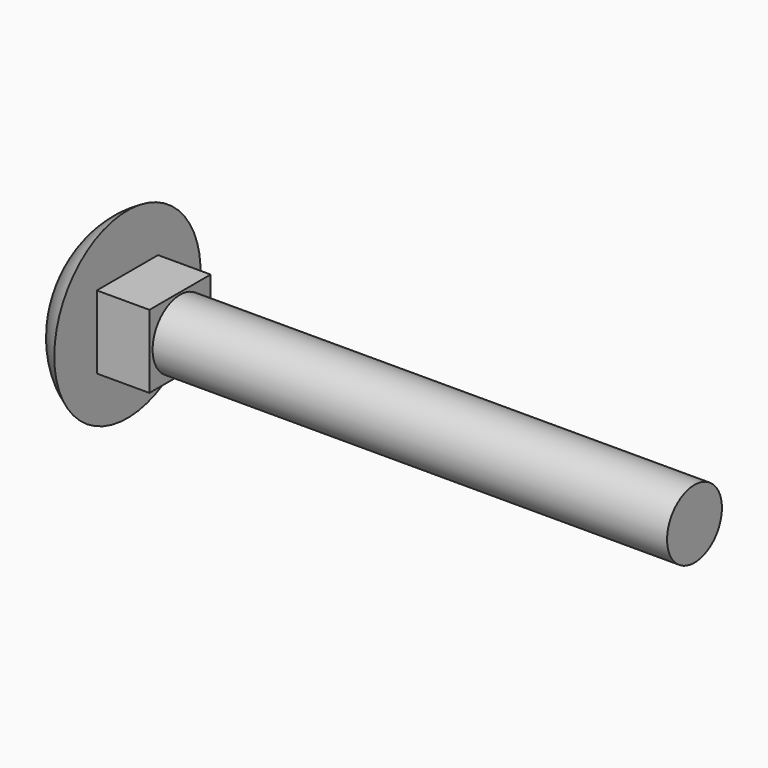
from build123d import *

# Parameters (mm, degrees)
F0_R     = 3
F1_DEPTH = 45
F2_W     = 3.3454523287
F2_H     = 3.2
F3_DEPTH = 4.6
F4_R     = 8
F5_DEPTH = 3.7


# Not quite as in the source:
# - a fillet or chamfer that OpenCascade refuses, or shapes differently, is made with other operations: its cross-section is extruded or revolved along the edge and cut away or added


with BuildPart() as f1:
    # F0 (on Right) → F1 (new body)
    with BuildSketch(Plane.YZ):
        Circle(F0_R)
    extrude(amount=F1_DEPTH)

    # F2 (on face) → F3 (join)
    with BuildSketch(Plane(origin=(0, 0, 0), x_dir=(0, -1, 0), z_dir=(-1, 0, 0))):
        with Locations((-1.6727261643, -1.6)):
            Rectangle(F2_W, F2_H)
        with Locations((-1.6727261643, 1.6)):
            Rectangle(F2_W, F2_H)
        Polygon((0, 3.2), (0, 0), (0, -3.2), (3.3454523287, -3.2), (3.3454523287, 0), (3.3454523287, 3.2), align=None)
    extrude(amount=F3_DEPTH)

    # F4 (on face) → F5 (join)
    with BuildSketch(Plane(origin=(-4.6, 0, 0), x_dir=(0, -1, 0), z_dir=(-1, 0, 0))):
        Circle(F4_R)
    extrude(amount=F5_DEPTH)

    # F6: fillet of radius 7 on 1 edges, made by hand

    # F6_s1 → F6_t2 (revolve, cut)
    with BuildSketch(Plane.XY):
        with BuildLine():
            ThreePointArc((-4.6, -8), (-7.3041652209, -5.4252811095), (-8.3, -1.8266702664))
            Line((-8.3, -1.8266702664), (-8.3, -8))
            Line((-8.3, -8), (-4.6, -8))
        make_face()
    revolve(axis=Axis((-8.3, 0, 0), (-1, 0, 0)), mode=Mode.SUBTRACT)


solid = f1.part
